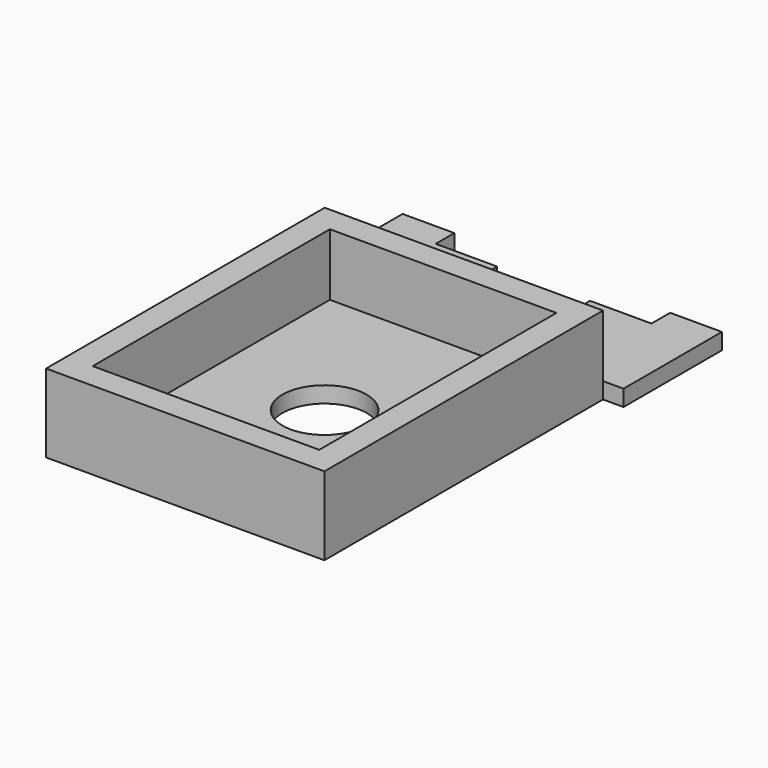
from build123d import *

# Parameters (mm, degrees)
F0_R     = 6.5
F1_DEPTH = 2.5
F3_DEPTH = 9.6


# Not quite as in the source:
# - a feature of the source that left no trace in its solid (it failed there, or was rolled back) is left out


with BuildPart() as f1:
    # F0 (on Top) → F1 (new body)
    with BuildSketch(Plane.XY):
        Polygon((-30.6198447943, 27.4039022624), (-27.4521095872, 27.4039022624), (-8.6198447943, 27.4039022624), (-8.6198447943, 35.4039022624), (-13.1198447943, 35.4039022624), (-13.1198447943, 42.8039022624), (-22.6198447943, 42.8039022624), (-22.6198447943, 46.4039022624), (-30.6198447943, 46.4039022624), align=None)
        Polygon((-3.2843746781, 35.4039022624), (-3.2843746781, 27.4039022624), (15.5478901148, 27.4039022624), (18.7156253219, 27.4039022624), (18.7156253219, 46.4039022624), (10.7156253219, 46.4039022624), (10.7156253219, 42.8039022624), (1.2156253219, 42.8039022624), (1.2156253219, 35.4039022624), align=None)
        Polygon((-8.6198447943, 27.4039022624), (-27.4521095872, 27.4039022624), (-27.4521095872, -26.3960977376), (-6.0521095872, -26.3960977376), (-5.8521098852, -26.3960977376), (15.5478901148, -26.3960977376), (15.5478901148, 27.4039022624), (-3.2843746781, 27.4039022624), (-5.8521098852, 27.4039022624), (-6.0521095872, 27.4039022624), align=None)
        Polygon((-23.4521095872, -22.3960977376), (-23.4521095872, 23.4039022624), (-5.9521097362, 23.4039022624), (11.5478901148, 23.4039022624), (11.5478901148, -22.3960977376), (-5.9521097362, -22.3960977376), align=None, mode=Mode.SUBTRACT)
        Polygon((-5.9521097362, 23.4039022624), (-23.4521095872, 23.4039022624), (-23.4521095872, -22.3960977376), (-5.9521097362, -22.3960977376), (11.5478901148, -22.3960977376), (11.5478901148, 23.4039022624), align=None)
        with Locations((-5.9521097362, 0.5039022624)):
            Circle(F0_R, mode=Mode.SUBTRACT)
    extrude(amount=-F1_DEPTH)

    # F0 (on Top) → F3 (join)
    with BuildSketch(Plane.XY):
        Polygon((-8.6198447943, 27.4039022624), (-27.4521095872, 27.4039022624), (-27.4521095872, -26.3960977376), (-6.0521095872, -26.3960977376), (-5.8521098852, -26.3960977376), (15.5478901148, -26.3960977376), (15.5478901148, 27.4039022624), (-3.2843746781, 27.4039022624), (-5.8521098852, 27.4039022624), (-6.0521095872, 27.4039022624), align=None)
        Polygon((-23.4521095872, -22.3960977376), (-23.4521095872, 23.4039022624), (-5.9521097362, 23.4039022624), (11.5478901148, 23.4039022624), (11.5478901148, -22.3960977376), (-5.9521097362, -22.3960977376), align=None, mode=Mode.SUBTRACT)
    extrude(amount=F3_DEPTH)


solid = f1.part
